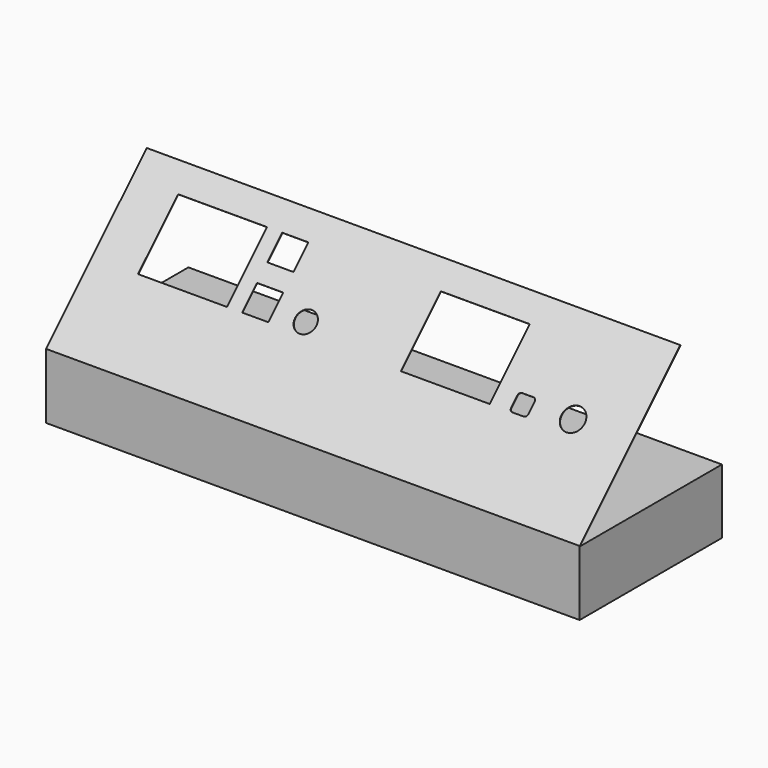
from build123d import *

# Parameters (mm, degrees)
F1_DEPTH = 209.55
F2_W     = 20.6375
F2_H     = 20.6375
F3_DEPTH = 0.4064


# Not quite as in the source:
# - the dataset's text gives a spline's control points without its knots; the knots are read off the source's solid


with BuildPart() as f1:
    # F0 (on Right) → F1 (new body, symmetric)
    with BuildSketch(Plane.YZ):
        Polygon((-139.7, 0), (0, 0), (0, 50.8), (-139.2936, 50.8), (-139.2936, 51.054), (-40.6298144724, 149.7177855276), (-40.9171826682, 150.0051537235), (-139.7, 51.2223363917), align=None)
    extrude(amount=F1_DEPTH, both=True)

    # F2 (on face) → F3 (cut, through all)
    with BuildSketch(Plane(origin=(0, -95.4611681959, 95.4611681959), x_dir=(1, 0, 0), z_dir=(0, -0.7071067812, 0.7071067812))):
        with BuildLine():
            add(Edge.make_bspline(
                [(119.0042372245, 14.038217476), (118.5632678245, 13.597959276), (118.3062706245, 12.977818276), (118.3062706245, 12.354959476)],
                knots=[1, 1, 1, 1, 2, 2, 2, 2], degree=3))
            Line((118.3062706245, 12.354959476), (118.3062706245, 3.623684076))
            add(Edge.make_bspline(
                [(118.3062706245, 3.623684076), (118.3062706245, 3.000114076), (118.5632678245, 2.380023876), (119.0042372245, 1.939740276)],
                knots=[0, 0, 0, 0, 1, 1, 1, 1], degree=3))
            add(Edge.make_bspline(
                [(119.0042372245, 1.939740276), (119.4445462245, 1.498770876), (120.0646618245, 1.242434076), (120.6875206245, 1.242434076)],
                knots=[1, 1, 1, 1, 2, 2, 2, 2], degree=3))
            Line((120.6875206245, 1.242434076), (129.4187706245, 1.242434076))
            add(Edge.make_bspline(
                [(129.4187706245, 1.242434076), (130.0423406245, 1.242434076), (130.6624562245, 1.498770876), (131.1027144245, 1.939740276)],
                knots=[0, 0, 0, 0, 1, 1, 1, 1], degree=3))
            add(Edge.make_bspline(
                [(131.1027144245, 1.939740276), (131.5436838245, 2.380023876), (131.8000206245, 3.000114076), (131.8000206245, 3.623684076)],
                knots=[1, 1, 1, 1, 2, 2, 2, 2], degree=3))
            Line((131.8000206245, 3.623684076), (131.8000206245, 12.354959476))
            add(Edge.make_bspline(
                [(131.8000206245, 12.354959476), (131.8000206245, 12.977818276), (131.5436838245, 13.597959276), (131.1027144245, 14.038217476)],
                knots=[0, 0, 0, 0, 1, 1, 1, 1], degree=3))
            add(Edge.make_bspline(
                [(131.1027144245, 14.038217476), (130.6624562245, 14.479186876), (130.0423406245, 14.736209476), (129.4187706245, 14.736209476)],
                knots=[1, 1, 1, 1, 2, 2, 2, 2], degree=3))
            Line((129.4187706245, 14.736209476), (120.6875206245, 14.736209476))
            add(Edge.make_bspline(
                [(120.6875206245, 14.736209476), (120.0646618245, 14.736209476), (119.4445462245, 14.479186876), (119.0042372245, 14.038217476)],
                knots=[0, 0, 0, 0, 1, 1, 1, 1], degree=3))
        make_face()
        Polygon((-173.3964987755, 56.804959476), (-173.3964987755, 1.242434076), (-103.5464987755, 1.242434076), (-103.5466765755, 56.804959476), align=None)
        Polygon((-91.6402487755, 1.242434076), (-71.0027487755, 1.242434076), (-71.0029265755, 21.879959476), (-91.6404265755, 21.879959476), align=None)
        with Locations((-81.3216765755, 46.486209476)):
            Rectangle(F2_W, F2_H)
        Polygon((32.9785012245, 1.242434076), (102.8281456245, 1.242434076), (102.8281456245, 56.804959476), (32.9781456245, 56.804959476), align=None)
        with BuildLine():
            add(Edge.make_bspline(
                [(-40.5029875755, 15.469304276), (-42.0462153755, 17.012709876), (-44.2145625755, 17.911209476), (-46.3966765755, 17.911209476)],
                knots=[7, 7, 7, 7, 8, 8, 8, 8], degree=3))
            add(Edge.make_bspline(
                [(-46.3966765755, 17.911209476), (-48.5784603755, 17.911209476), (-50.7468075755, 17.012709876), (-52.2898575755, 15.469304276)],
                knots=[0, 0, 0, 0, 1, 1, 1, 1], degree=3))
            add(Edge.make_bspline(
                [(-52.2898575755, 15.469304276), (-53.8329075755, 13.926609876), (-54.7310515755, 11.758262676), (-54.7310515755, 9.576834476), (-54.7310515755, 7.394720476), (-53.8327297755, 5.226373276), (-52.2896797755, 3.682967676)],
                knots=[1, 1, 1, 1, 2, 2, 2, 3, 3, 3, 3], degree=3))
            add(Edge.make_bspline(
                [(-52.2896797755, 3.682967676), (-50.7466297755, 2.140222476), (-48.5782825755, 1.242434076), (-46.3964987755, 1.242434076), (-44.2143847755, 1.242434076), (-42.0460375755, 2.140222476), (-40.5029875755, 3.682967676)],
                knots=[3, 3, 3, 3, 4, 4, 4, 5, 5, 5, 5], degree=3))
            add(Edge.make_bspline(
                [(-40.5029875755, 3.682967676), (-38.9602677755, 5.226373276), (-38.0624793755, 7.394720476), (-38.0624793755, 9.576834476), (-38.0624793755, 11.758262676), (-38.9602677755, 13.926609876), (-40.5029875755, 15.469304276)],
                knots=[5, 5, 5, 5, 6, 6, 6, 7, 7, 7, 7], degree=3))
        make_face()
        with BuildLine():
            add(Edge.make_bspline(
                [(169.6082508245, 16.824597476), (167.9183888245, 18.514789676), (165.5433618245, 19.498709476), (163.1535012245, 19.498709476)],
                knots=[7, 7, 7, 7, 8, 8, 8, 8], degree=3))
            add(Edge.make_bspline(
                [(163.1535012245, 19.498709476), (160.7636406245, 19.498709476), (158.3889184245, 18.514789676), (156.6991072245, 16.824597476)],
                knots=[0, 0, 0, 0, 1, 1, 1, 1], degree=3))
            add(Edge.make_bspline(
                [(156.6991072245, 16.824597476), (155.0092706245, 15.135141876), (154.0253762245, 12.760114876), (154.0253762245, 10.370584476), (154.0253762245, 7.980368276), (155.0092706245, 5.605315876), (156.6991072245, 3.915834876)],
                knots=[1, 1, 1, 1, 2, 2, 2, 3, 3, 3, 3], degree=3))
            add(Edge.make_bspline(
                [(156.6991072245, 3.915834876), (158.3889184245, 2.225668076), (160.7636406245, 1.242434076), (163.1535012245, 1.242434076), (165.5433618245, 1.242434076), (167.9183888245, 2.225668076), (169.6082508245, 3.915834876)],
                knots=[3, 3, 3, 3, 4, 4, 4, 5, 5, 5, 5], degree=3))
            add(Edge.make_bspline(
                [(169.6082508245, 3.915834876), (171.2980366245, 5.605315876), (172.2816262245, 7.980368276), (172.2816262245, 10.370584476), (172.2816262245, 12.760114876), (171.2980366245, 15.135141876), (169.6082508245, 16.824597476)],
                knots=[5, 5, 5, 5, 6, 6, 6, 7, 7, 7, 7], degree=3))
        make_face()
    extrude(amount=-F3_DEPTH, mode=Mode.SUBTRACT)


solid = f1.part
